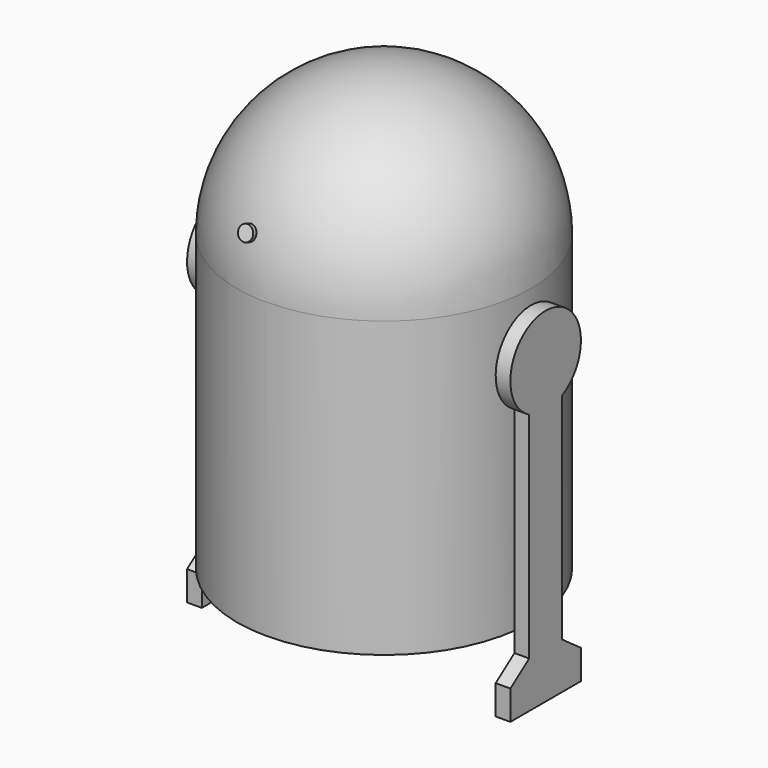
from build123d import *
from build123d import SkipClean  # not in build123d's __all__

# Parameters (mm, degrees)
F0_R      = 63.5
F1_DEPTH  = 127
F6_DEPTH  = 6.35
F10_R     = 3.175
F11_DEPTH = 64.77


with BuildPart() as f1:
    # F0 (on Top) → F1 (new body)
    with BuildSketch(Plane.XY):
        Circle(F0_R)
    extrude(amount=F1_DEPTH)

    # F2 (on face) → F3 (revolve)
    with BuildSketch(Plane.XY.offset(127)):
        with BuildLine():
            Line((0, -63.5), (0, 63.5))
            ThreePointArc((0, 63.5), (-63.5, 0), (0, -63.5))
        make_face()
    with SkipClean():  # cleaning this boolean's faces spoils the solid; the shape is the same uncleaned
        revolve(axis=Axis((0, 0, 127), (0, -1, 0)))


with BuildPart() as f6:
    # F5 (on offset) → F6 (new body)
    with BuildSketch(Plane.YZ.offset(63.5)):
        with BuildLine():
            ThreePointArc((8.89, 84.751546065), (16.3134453749, 91.7626223006), (19.05, 101.6))
            ThreePointArc((19.05, 101.6), (-9.8373776994, 117.9134453749), (-8.89, 84.751546065))
            ThreePointArc((-8.89, 84.751546065), (0, 82.55), (8.89, 84.751546065))
        make_face()
        with BuildLine():
            ThreePointArc((8.89, 84.751546065), (0, 82.55), (-8.89, 84.751546065))
            Line((-8.89, 84.751546065), (-8.89, -8.0432999057))
            Line((-8.89, -8.0432999057), (-19.05, -15.3457973657))
            Line((-19.05, -15.3457973657), (-19.05, -28.0457973657))
            Line((-19.05, -28.0457973657), (19.05, -28.0457973657))
            Line((19.05, -28.0457973657), (19.05, -15.3457973657))
            Line((19.05, -15.3457973657), (8.89, -8.0432999057))
            Line((8.89, -8.0432999057), (8.89, 84.751546065))
        make_face()
    extrude(amount=F6_DEPTH)


with BuildPart() as f7_1:
    # F7: instance of F6
    add(f6.part.mirror(Plane.YZ), clean=False)


with BuildPart() as f11:
    # F10 (on line) → F11 (new body)
    with BuildSketch(Plane(origin=(0, -40.8170132151, 14.8561778619), x_dir=(1, 0, 0), z_dir=(0, -0.9396926208, 0.3420201433))):
        with Locations((-10.9879607335, 118.8522130251)):
            Circle(F10_R)
    extrude(amount=F11_DEPTH)


solid = Compound([f1.part, f6.part, f7_1.part, f11.part])
